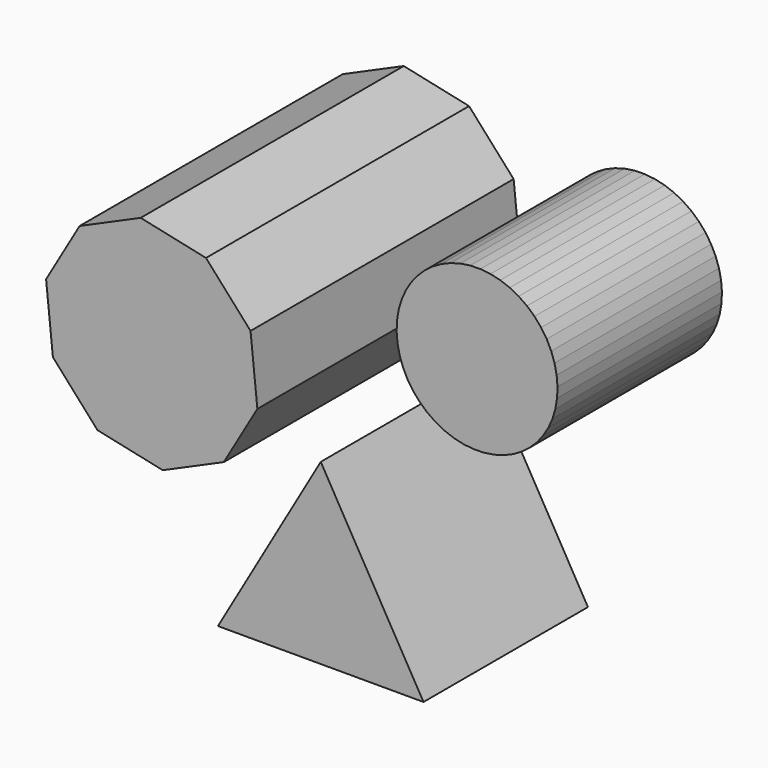
from build123d import *

# Parameters (mm, degrees)
F1_DEPTH = 50
F3_DEPTH = 80
F5_DEPTH = 50


# Not quite as in the source:
# - the program builds the solid bodies; features that only make, move or delete a surface that nothing else refers to are left out


with BuildPart() as f1:
    # F0 (on Front) → F1 (new body)
    with BuildSketch(Plane.XZ):
        Polygon((-25, 14.3545279566), (-50, -28.9467422326), (0, -28.9467422326), align=None)
    extrude(amount=F1_DEPTH)


with BuildPart() as f3:
    # F2 (on Front) → F3 (new body)
    with BuildSketch(Plane.XZ):
        Polygon((-24.5748425958, 26.6332762849), (-16.4171555915, 40.6826237873), (-18.0754474364, 56.8437527904), (-28.9163070091, 68.9436613118), (-44.79889442, 72.360595557), (-59.6566011074, 65.7894027817), (-67.8142881117, 51.7400552794), (-66.1559962667, 35.5789262762), (-55.3151366941, 23.4790177548), (-39.4325492832, 20.0620835096), align=None)
    extrude(amount=F3_DEPTH)


with BuildPart() as f5:
    # F4 (on Front) → F5 (new body)
    with BuildSketch(Plane.XZ):
        Polygon((30.3777791232, 39.6685771282), (31.3758142621, 41.9141553704), (32.0845340135, 44.2671135286), (32.4927614435, 46.6903440471), (32.5940585619, 49.145631133), (32.3868278523, 51.5942534423), (31.874337467, 53.9975947383), (31.0646696855, 56.3177528933), (29.9705934524, 58.518137627), (28.6093630033, 60.5640475578), (27.0024457557, 62.4232174639), (25.1751837545, 64.0663271253), (23.156394013, 65.467463721), (20.9779140514, 66.60453049), (18.6740998, 67.4595952101), (16.2812837859, 68.0191729998), (13.8372021469, 68.2744389831), (11.3803995105, 68.2213674629), (8.9496211219, 67.8607954089), (6.5832018085, 67.1984092578), (4.3184614163, 66.2446552347), (2.1911162543, 65.0145746105), (0.2347158265, 63.5275664914), (-1.5198862636, 61.8070818836), (-3.0450188931, 59.8802538573), (-4.3166298091, 57.7774696414), (-5.314664948, 55.5318913992), (-6.0233846994, 53.178933241), (-6.4316121295, 50.7557027225), (-6.5329092478, 48.3004156366), (-6.3256785383, 45.8517933273), (-5.813188153, 43.4484520313), (-5.0035203715, 41.1282938764), (-3.9094441383, 38.9279091426), (-2.5482136893, 36.8819992118), (-0.9412964417, 35.0228293057), (0.8859655595, 33.3797196443), (2.904755301, 31.9785830486), (5.0832352626, 30.8415162796), (7.387049514, 29.9864515595), (9.7798655282, 29.4268737698), (12.2239471672, 29.1716077865), (14.6807498036, 29.2246793067), (17.1115281921, 29.5852513607), (19.4779475056, 30.2476375118), (21.7426878977, 31.2013915349), (23.8700330597, 32.4314721591), (25.8264334875, 33.9184802783), (27.5810355777, 35.638964886), (29.1061682071, 37.5657929123), align=None)
    extrude(amount=F5_DEPTH)


solid = Compound([f1.part, f3.part, f5.part])
